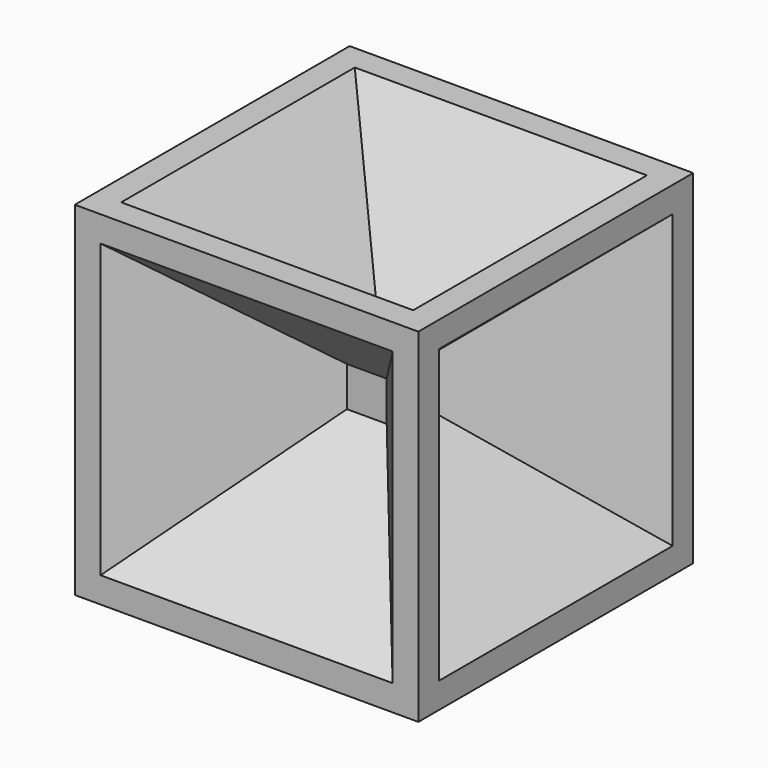
from build123d import *

# Parameters (mm, degrees)
F0_W           = 101.6
F0_H           = 101.6
F1_DEPTH       = 101.6
F2_W           = 86.36
F2_H           = 86.36
F3_DEPTH       = 46.99
F3_TAPER       = 40
F4_W           = 86.36
F4_H           = 86.36
F5_DEPTH       = 46.99
F5_TAPER       = 40
F6_W           = 86.36
F6_H           = 86.36
F7_DEPTH       = 46.99
F7_TAPER       = 40
F8_W           = 86.36
F8_H           = 86.36
F9_DEPTH       = 46.99
F9_TAPER       = 40
F10_W          = 86.36
F10_H          = 86.36
F11_DEPTH      = 46.99
F11_TAPER      = 40
F12_W          = 86.36
F12_H          = 86.36
F13_DEPTH      = 46.99
F13_TAPER      = 40
F14_W          = 12.581416662
F14_H          = 12.581416662
F15_DEPTH      = 2.54
F15_DEPTH_BACK = 10.16


with BuildPart() as f1:
    # F0 (on Top) → F1 (new body)
    with BuildSketch(Plane.XY):
        with Locations((-50.8, 50.8)):
            Rectangle(F0_W, F0_H)
    extrude(amount=F1_DEPTH)

    # F2 (on face) → F3 (cut)
    with BuildSketch(Plane.XZ):
        with Locations((-50.8, 50.8)):
            Rectangle(F2_W, F2_H)
    extrude(amount=-F3_DEPTH, taper=F3_TAPER, mode=Mode.SUBTRACT)

    # F4 (on face) → F5 (cut)
    with BuildSketch(Plane.YZ):
        with Locations((50.8, 50.8)):
            Rectangle(F4_W, F4_H)
    extrude(amount=-F5_DEPTH, taper=F5_TAPER, mode=Mode.SUBTRACT)

    # F6 (on face) → F7 (cut)
    with BuildSketch(Plane.XY.offset(101.6)):
        with Locations((-50.8, 50.8)):
            Rectangle(F6_W, F6_H)
    extrude(amount=-F7_DEPTH, taper=F7_TAPER, mode=Mode.SUBTRACT)

    # F8 (on face) → F9 (cut)
    with BuildSketch(Plane(origin=(-101.6, 0, 0), x_dir=(0, -1, 0), z_dir=(-1, 0, 0))):
        with Locations((-50.8, 50.8)):
            Rectangle(F8_W, F8_H)
    extrude(amount=-F9_DEPTH, taper=F9_TAPER, mode=Mode.SUBTRACT)

    # F10 (on face) → F11 (cut)
    with BuildSketch(Plane(origin=(0, 101.6, 0), x_dir=(-1, 0, 0), z_dir=(0, 1, 0))):
        with Locations((50.8, 50.8)):
            Rectangle(F10_W, F10_H)
    extrude(amount=-F11_DEPTH, taper=F11_TAPER, mode=Mode.SUBTRACT)

    # F12 (on face) → F13 (cut)
    with BuildSketch(Plane(origin=(0, 0, 0), x_dir=(1, 0, 0), z_dir=(0, 0, -1))):
        with Locations((-50.8, -50.8)):
            Rectangle(F12_W, F12_H)
    extrude(amount=-F13_DEPTH, taper=F13_TAPER, mode=Mode.SUBTRACT)

    # F14 (on face) → F15 (join, two sides)
    with BuildSketch(Plane.XZ.offset(-46.99)) as f15_sk:
        with Locations((-50.8, 50.8)):
            Rectangle(F14_W, F14_H)
    extrude(amount=F15_DEPTH)
    extrude(f15_sk.sketch, amount=-F15_DEPTH_BACK)


solid = f1.part
